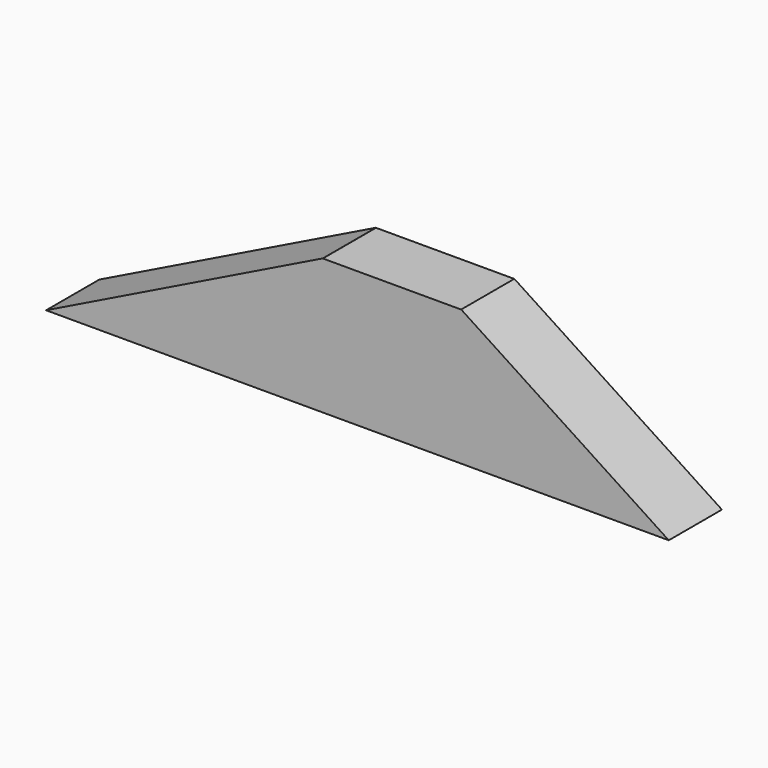
from build123d import *

# Parameters (mm, degrees)
F0_W     = 100
F0_H     = 98
F1_DEPTH = 48


# Not quite as in the source:
# - a feature names something its author has since deleted; it is built from what else it names


with BuildPart() as f1:
    # F0 (on Front) → F1 (new body)
    with BuildSketch(Plane.XZ):
        Rectangle(F0_W, F0_H)
        Polygon((-250, -49), (-50, -49), (-50, 49), (-50, 49.0569584072), align=None)
        Polygon((50, 49), (50, -49), (200, -49), (50, 49.0569546819), align=None)
    extrude(amount=F1_DEPTH)


solid = f1.part
